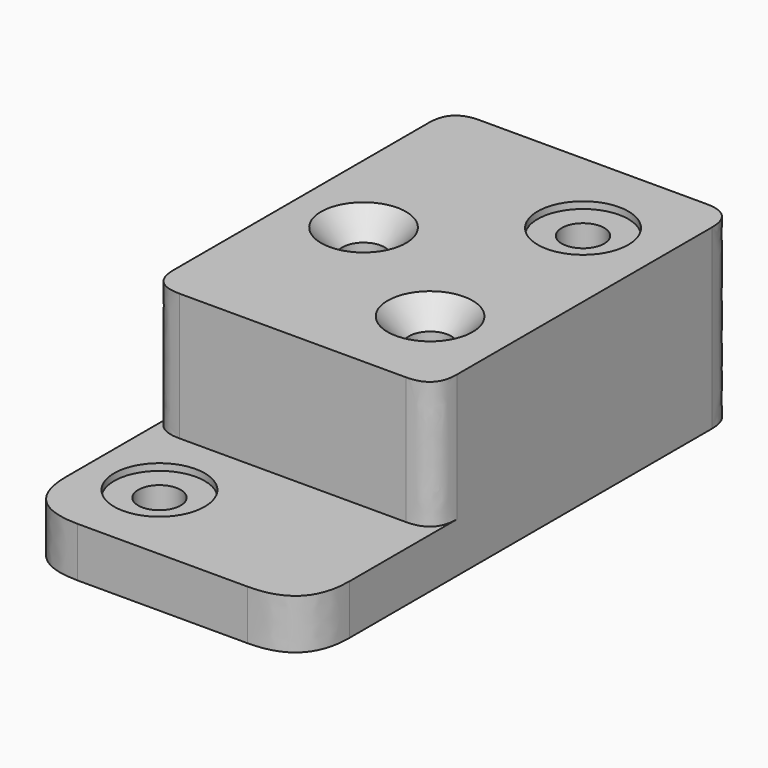
from build123d import *

# Parameters (mm, degrees)
F0_W           = 127
F0_H           = 22.352
F1_DEPTH       = 241.3
F2_W           = 127
F2_H           = 168.402
F3_DEPTH       = 57.15
F5_D           = 19.05
F5_CSINK_D     = 38.1
F5_CSINK_ANGLE = 82
F6_D           = 19.05
F6_START       = 57.15
F6_CBORE_D     = 40.64
F6_CBORE_DEPTH = 3.048
F7_T1_DEPTH    = 149.352
F8_T1_DEPTH    = 88.9
F9_T1_DEPTH    = 88.9
F10_T1_DEPTH   = 149.352
F11_T1_DEPTH   = 143.002
F12_T1_DEPTH   = 143.002


# Not quite as in the source:
# - a fillet or chamfer that OpenCascade refuses, or shapes differently, is made with other operations: its cross-section is extruded or revolved along the edge and cut away or added


with BuildPart() as f1:
    # F0 (on Front) → F1 (new body)
    with BuildSketch(Plane.XZ):
        with Locations((63.5, 11.176)):
            Rectangle(F0_W, F0_H)
    extrude(amount=-F1_DEPTH)

    # F2 (on face) → F3 (join)
    with BuildSketch(Plane.XY.offset(22.352)):
        with Locations((63.5, 157.099)):
            Rectangle(F2_W, F2_H)
    extrude(amount=F3_DEPTH)

    # F5 (through all)
    with Locations(Plane.XY.offset(79.502)):
        with Locations((31.75, 152.4), (92.075, 114.3)):
            CounterSinkHole(F5_D / 2, F5_CSINK_D / 2, counter_sink_angle=F5_CSINK_ANGLE)

    # F6 (through all)
    # its depths count from where the whole tool has entered the part; down to there all is cleared
    with Locations(Plane.XY.offset(79.502)):
        with Locations((92.075, 200.025, 0), (31.75, 37.973, -F6_START)):
            CounterBoreHole(F6_D / 2, F6_CBORE_D / 2, F6_CBORE_DEPTH)

    # F7: fillet of radius 25.4 on 1 edges, made by hand

    # F7_s2 → F7_t1 (cut)
    with BuildSketch(Plane.XY.offset(-63.5)):
        with BuildLine():
            add(Edge.make_bspline(
                [(101.6, 0), (127, 0), (127, 25.4)],
                knots=[0, 0, 0, 1, 1, 1], degree=2, weights=[1, 1, 1]))
            Line((127, 25.4), (127, 0))
            Line((127, 0), (101.6, 0))
        make_face()
    extrude(amount=F7_T1_DEPTH, mode=Mode.SUBTRACT)

    # F8: fillet of radius 12.7 on 1 edges, made by hand

    # F8_s2 → F8_t1 (cut)
    with BuildSketch(Plane.XY.offset(22.352)):
        with BuildLine():
            add(Edge.make_bspline(
                [(114.3, 72.898), (127, 72.898), (127, 85.598)],
                knots=[0, 0, 0, 1, 1, 1], degree=2, weights=[1, 1, 1]))
            Line((127, 85.598), (127, 72.898))
            Line((127, 72.898), (114.3, 72.898))
        make_face()
    extrude(amount=F8_T1_DEPTH, mode=Mode.SUBTRACT)

    # F9: fillet of radius 12.7 on 1 edges, made by hand

    # F9_s2 → F9_t1 (cut)
    with BuildSketch(Plane.XY.offset(22.352)):
        with BuildLine():
            add(Edge.make_bspline(
                [(0, 85.598), (0, 72.898), (12.7, 72.898)],
                knots=[0, 0, 0, 1, 1, 1], degree=2, weights=[1, 1, 1]))
            Line((12.7, 72.898), (0, 72.898))
            Line((0, 72.898), (0, 85.598))
        make_face()
    extrude(amount=F9_T1_DEPTH, mode=Mode.SUBTRACT)

    # F10: fillet of radius 25.4 on 1 edges, made by hand

    # F10_s2 → F10_t1 (cut)
    with BuildSketch(Plane.XY.offset(-63.5)):
        with BuildLine():
            add(Edge.make_bspline(
                [(0, 25.4), (0, 0), (25.4, 0)],
                knots=[0, 0, 0, 1, 1, 1], degree=2, weights=[1, 1, 1]))
            Line((25.4, 0), (0, 0))
            Line((0, 0), (0, 25.4))
        make_face()
    extrude(amount=F10_T1_DEPTH, mode=Mode.SUBTRACT)

    # F11: fillet of radius 12.7 on 1 edges, made by hand

    # F11_s2 → F11_t1 (cut)
    with BuildSketch(Plane.XY.offset(-31.75)):
        with BuildLine():
            add(Edge.make_bspline(
                [(114.3, 241.3), (127, 241.3), (127, 228.6)],
                knots=[0, 0, 0, 1, 1, 1], degree=2, weights=[1, 1, 1]))
            Line((127, 228.6), (127, 241.3))
            Line((127, 241.3), (114.3, 241.3))
        make_face()
    extrude(amount=F11_T1_DEPTH, mode=Mode.SUBTRACT)

    # F12: fillet of radius 12.7 on 1 edges, made by hand

    # F12_s2 → F12_t1 (cut)
    with BuildSketch(Plane.XY.offset(-31.75)):
        with BuildLine():
            add(Edge.make_bspline(
                [(0, 228.6), (0, 241.3), (12.7, 241.3)],
                knots=[0, 0, 0, 1, 1, 1], degree=2, weights=[1, 1, 1]))
            Line((12.7, 241.3), (0, 241.3))
            Line((0, 241.3), (0, 228.6))
        make_face()
    extrude(amount=F12_T1_DEPTH, mode=Mode.SUBTRACT)


solid = f1.part
